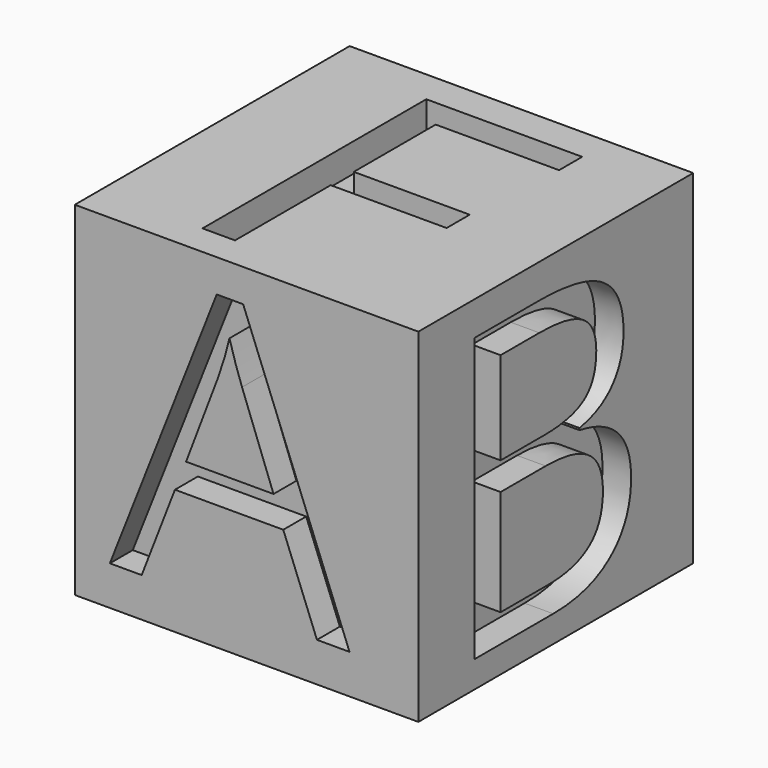
from build123d import *

# Parameters (mm, degrees)
F0_W          = 76.2
F0_H          = 76.2
F1_DEPTH      = 76.2
F2_TEXT_SIZE  = 83.9898233405
F3_DEPTH      = 6.35
F4_TEXT_SIZE  = 87.8662763474
F5_DEPTH      = 6.35
F6_TEXT_SIZE  = 86.8971627723
F7_DEPTH      = 6.35
F8_TEXT_SIZE  = 84.3128668041
F9_DEPTH      = 6.35
F10_TEXT_SIZE = 86.2510933075
F11_DEPTH     = 6.35
F12_TEXT_SIZE = 86.8971653593
F13_DEPTH     = 6.35


# Not quite as in the source:
# - Text() gives the source's letters only with a copy of the font that has no kerning and outlines rounded to 1/6400 em; it was checked with that copy


with BuildPart() as f1:
    # F0 (on Front) → F1 (new body)
    with BuildSketch(Plane.XZ):
        with Locations((-12.2406412899, 24.9676587939)):
            Rectangle(F0_W, F0_H)
    extrude(amount=F1_DEPTH)

    # F2 (on face) → F3 (cut)
    with BuildSketch(Plane.XZ.offset(76.2)):
        with Locations((-42.5634607673, -4.4191572815)):
            Text('A', F2_TEXT_SIZE, font='Open Sans', text_align=(TextAlign.LEFT, TextAlign.BOTTOM))
    extrude(amount=-F3_DEPTH, mode=Mode.SUBTRACT)

    # F4 (on face) → F5 (cut)
    with BuildSketch(Plane.YZ.offset(25.8593587101)):
        with Locations((-69.3109929562, -7.2102034464)):
            Text('B', F4_TEXT_SIZE, font='Open Sans', text_align=(TextAlign.LEFT, TextAlign.BOTTOM))
    extrude(amount=-F5_DEPTH, mode=Mode.SUBTRACT)

    # F6 (on face) → F7 (cut)
    with BuildSketch(Plane(origin=(0, 0, 0), x_dir=(-1, 0, 0), z_dir=(0, 1, 0))):
        with Locations((-17.4440406263, -5.8146798983)):
            Text('C', F6_TEXT_SIZE, font='Open Sans', text_align=(TextAlign.LEFT, TextAlign.BOTTOM))
    extrude(amount=-F7_DEPTH, mode=Mode.SUBTRACT)

    # F8 (on face) → F9 (cut)
    with BuildSketch(Plane(origin=(-50.3406412899, 0, 0), x_dir=(0, -1, 0), z_dir=(-1, 0, 0))):
        with Locations((8.140552789, -5.8146798983)):
            Text('D', F8_TEXT_SIZE, font='Open Sans', text_align=(TextAlign.LEFT, TextAlign.BOTTOM))
    extrude(amount=-F9_DEPTH, mode=Mode.SUBTRACT)

    # F10 (on face) → F11 (cut)
    with BuildSketch(Plane(origin=(0, 0, -13.1323412061), x_dir=(1, 0, 0), z_dir=(0, 0, -1))):
        with Locations((-41.8656989932, 7.4427905492)):
            Text('E', F10_TEXT_SIZE, font='Open Sans', text_align=(TextAlign.LEFT, TextAlign.BOTTOM))
    extrude(amount=-F11_DEPTH, mode=Mode.SUBTRACT)

    # F12 (on face) → F13 (cut)
    with BuildSketch(Plane.XY.offset(63.0676587939)):
        with Locations((-36.0510181636, -69.3109882995)):
            Text('F', F12_TEXT_SIZE, font='Open Sans', text_align=(TextAlign.LEFT, TextAlign.BOTTOM))
    extrude(amount=-F13_DEPTH, mode=Mode.SUBTRACT)


solid = f1.part
